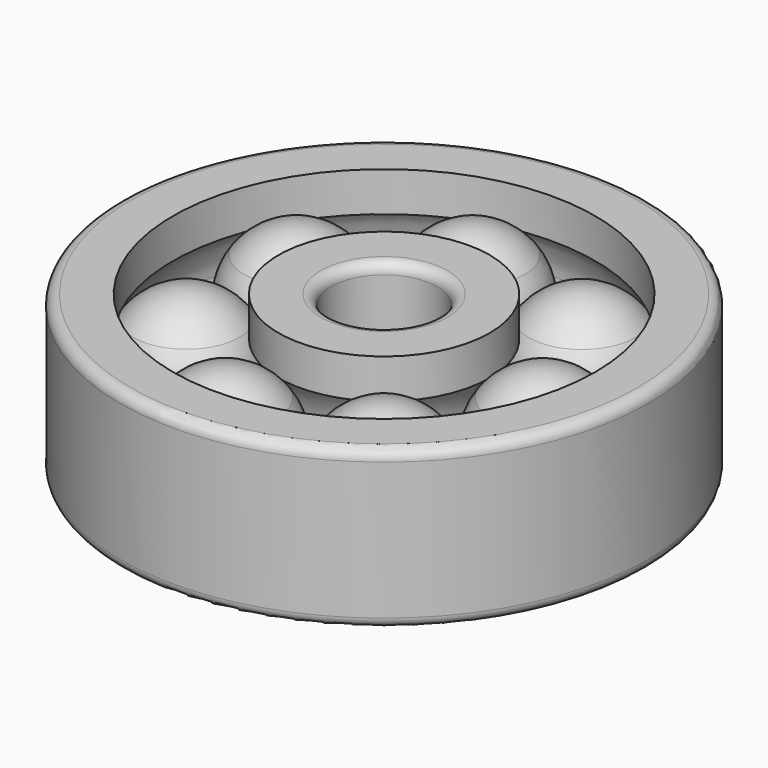
from build123d import *

# Parameters (mm, degrees)
F3_COUNT = 7
F4_R     = 2.54
F4_2_R   = 2.54


with BuildPart() as f1:
    # F0 (on Front) → F1 (revolve)
    with BuildSketch(Plane.XZ):
        with BuildLine():
            Line((50.8, 19.05), (50.8, 9.525))
            ThreePointArc((50.8, 9.525), (53.1603473566, 5.0201157855), (53.975, 0))
            ThreePointArc((53.975, 0), (53.1603473566, -5.0201157855), (50.8, -9.525))
            Line((50.8, -9.525), (50.8, -19.05))
            Line((50.8, -19.05), (63.5, -19.05))
            Line((63.5, -19.05), (63.5, 19.05))
            Line((63.5, 19.05), (50.8, 19.05))
        make_face()
    revolve(axis=Axis((0, 0, -3.4924996912), (0, 0, -1)))

    # F4
    f4_edges = [f1.edges().sort_by_distance(p)[0] for p in [
        (-63.5, 0, 19.05),
        (-63.5, 0, -19.05),
    ]]
    fillet(f4_edges, radius=F4_R)


with BuildPart() as f1b:
    # F0 (on Front) → F1, piece 2 (revolve)
    with BuildSketch(Plane.XZ):
        with BuildLine():
            Line((25.4, 19.05), (12.7, 19.05))
            Line((12.7, 19.05), (12.7, -19.05))
            Line((12.7, -19.05), (25.4, -19.05))
            Line((25.4, -19.05), (25.4, -9.525))
            ThreePointArc((25.4, -9.525), (22.225, 0), (25.4, 9.525))
            Line((25.4, 9.525), (25.4, 19.05))
        make_face()
    revolve(axis=Axis((0, 0, -3.4924996912), (0, 0, -1)))

    # F4#2
    f4_2_edges = [f1b.edges().sort_by_distance(p)[0] for p in [
        (-12.7, 0, 19.05),
        (-12.7, 0, -19.05),
    ]]
    fillet(f4_2_edges, radius=F4_2_R)


with BuildPart() as f2:
    # F0 (on Front) → F2 (revolve)
    with BuildSketch(Plane.XZ):
        with BuildLine():
            ThreePointArc((50.8, 9.525), (45.1995158286, 14.1990316571), (38.1, 15.875))
            Line((38.1, 15.875), (38.1, -15.875))
            ThreePointArc((38.1, -15.875), (45.1995158286, -14.1990316571), (50.8, -9.525))
            Line((50.8, -9.525), (50.8, 9.525))
        make_face()
        with BuildLine():
            ThreePointArc((53.975, 0), (53.1603473566, 5.0201157855), (50.8, 9.525))
            Line((50.8, 9.525), (50.8, -9.525))
            ThreePointArc((50.8, -9.525), (53.1603473566, -5.0201157855), (53.975, 0))
        make_face()
    revolve(axis=Axis((38.1, 0, 0), (0, 0, -1)))


with BuildPart() as f3_1:
    # F3: instance of F2
    add(f2.part.rotate(Axis((0, 0, -3.4924996912), (0, 0, -1)), 1 * 360 / F3_COUNT))


with BuildPart() as f3_2:
    # F3: instance of F2
    add(f2.part.rotate(Axis((0, 0, -3.4924996912), (0, 0, -1)), 2 * 360 / F3_COUNT))


with BuildPart() as f3_3:
    # F3: instance of F2
    add(f2.part.rotate(Axis((0, 0, -3.4924996912), (0, 0, -1)), 3 * 360 / F3_COUNT))


with BuildPart() as f3_4:
    # F3: instance of F2
    add(f2.part.rotate(Axis((0, 0, -3.4924996912), (0, 0, -1)), 4 * 360 / F3_COUNT))


with BuildPart() as f3_5:
    # F3: instance of F2
    add(f2.part.rotate(Axis((0, 0, -3.4924996912), (0, 0, -1)), 5 * 360 / F3_COUNT))


with BuildPart() as f3_6:
    # F3: instance of F2
    add(f2.part.rotate(Axis((0, 0, -3.4924996912), (0, 0, -1)), 6 * 360 / F3_COUNT))


solid = Compound([f1.part, f1b.part, f2.part, f3_1.part, f3_2.part, f3_3.part, f3_4.part, f3_5.part, f3_6.part])
